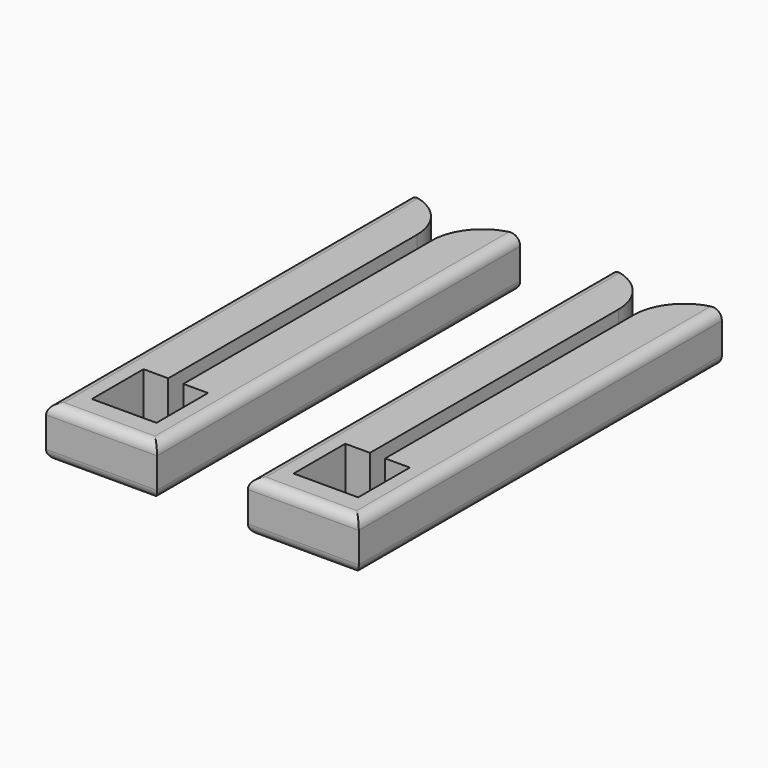
from build123d import *

# Parameters (mm, degrees)
F0_W        = 11
F0_H        = 45
F0_W_2      = 6.4
F0_H_2      = 6.4
F1_DEPTH    = 5
F2_W        = 1.5
F2_H        = 10
F3_DEPTH    = 37
F4_T1_DEPTH = 29.9687304443
F5_R        = 1


# Not quite as in the source:
# - a fillet or chamfer that OpenCascade refuses, or shapes differently, is made with other operations: its cross-section is extruded or revolved along the edge and cut away or added


with BuildPart() as f1:
    # F0 (on Top) → F1 (new body)
    with BuildSketch(Plane.XY):
        Rectangle(F0_W, F0_H)
        with Locations((0, -16.5)):
            Rectangle(F0_W_2, F0_H_2, mode=Mode.SUBTRACT)
    extrude(amount=F1_DEPTH)

    # F2 (on face) → F3 (cut)
    with BuildSketch(Plane(origin=(0, 22.5, 0), x_dir=(-1, 0, 0), z_dir=(0, 1, 0))):
        with Locations((0, 5)):
            Rectangle(F2_W, F2_H)
    extrude(amount=-F3_DEPTH, mode=Mode.SUBTRACT)

    # F4: fillet of radius 5 on 2 edges, made by hand

    # F4_s2 → F4_t1 (cut)
    with BuildSketch(Plane.XY.offset(-12.4843652221)):
        with BuildLine():
            ThreePointArc((-5.5, 22.5), (-2.1271558135, 20.9522660992), (-0.75, 17.5062539111))
            Line((-0.75, 17.5062539111), (-0.75, 22.5))
            Line((-0.75, 22.5), (-5.5, 22.5))
        make_face()
        with BuildLine():
            ThreePointArc((5.5, 22.5), (2.1271558135, 20.9522660992), (0.75, 17.5062539111))
            Line((0.75, 17.5062539111), (0.75, 22.5))
            Line((0.75, 22.5), (5.5, 22.5))
        make_face()
    extrude(amount=F4_T1_DEPTH, mode=Mode.SUBTRACT)

    # F5
    f5_edges = [f1.edges().sort_by_distance(p)[0] for p in [
        (-5.5, 0, 5),
        (5.5, 0, 5),
        (5.5, 0, 0),
        (-5.5, 0, 0),
        (0, -22.5, 5),
        (0, -22.5, 0),
    ]]
    fillet(f5_edges, radius=F5_R)


with BuildPart() as f6_1:
    # F6: copy of F1
    add(f1.part.moved(Location((20, 0, 0))))


solid = Compound([f1.part, f6_1.part])
